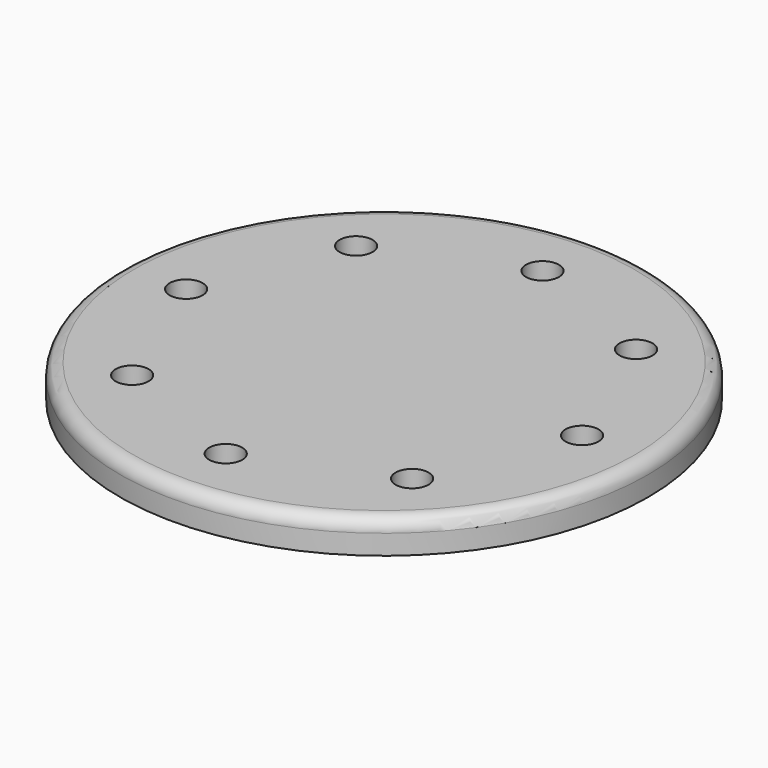
from build123d import *

# Parameters (mm, degrees)
F0_R     = 50.8
F0_R_2   = 3.175
F1_DEPTH = 6.35
F10_R    = 2.54


# Not quite as in the source:
# - the program builds the solid bodies; features that only make, move or delete a surface that nothing else refers to are left out


with BuildPart() as f1:
    # F0 (on Top) → F1 (new body)
    with BuildSketch(Plane.XY):
        Circle(F0_R)
        with Locations((-26.9407683632, -26.9407683632)):
            Circle(F0_R_2, mode=Mode.SUBTRACT)
        with Locations((0, -38.1)):
            Circle(F0_R_2, mode=Mode.SUBTRACT)
        with Locations((-38.1, 0)):
            Circle(F0_R_2, mode=Mode.SUBTRACT)
        with Locations((26.9407683632, -26.9407683632)):
            Circle(F0_R_2, mode=Mode.SUBTRACT)
        with Locations((38.1, 0)):
            Circle(F0_R_2, mode=Mode.SUBTRACT)
        with Locations((-26.9407683632, 26.9407683632)):
            Circle(F0_R_2, mode=Mode.SUBTRACT)
        with Locations((0, 38.1)):
            Circle(F0_R_2, mode=Mode.SUBTRACT)
        with Locations((26.9407683632, 26.9407683632)):
            Circle(F0_R_2, mode=Mode.SUBTRACT)
    extrude(amount=F1_DEPTH)

    # F10
    f10_edges = [f1.edges().sort_by_distance(p)[0] for p in [
        (-50.8, 0, 6.35),
    ]]
    fillet(f10_edges, radius=F10_R)


solid = f1.part
